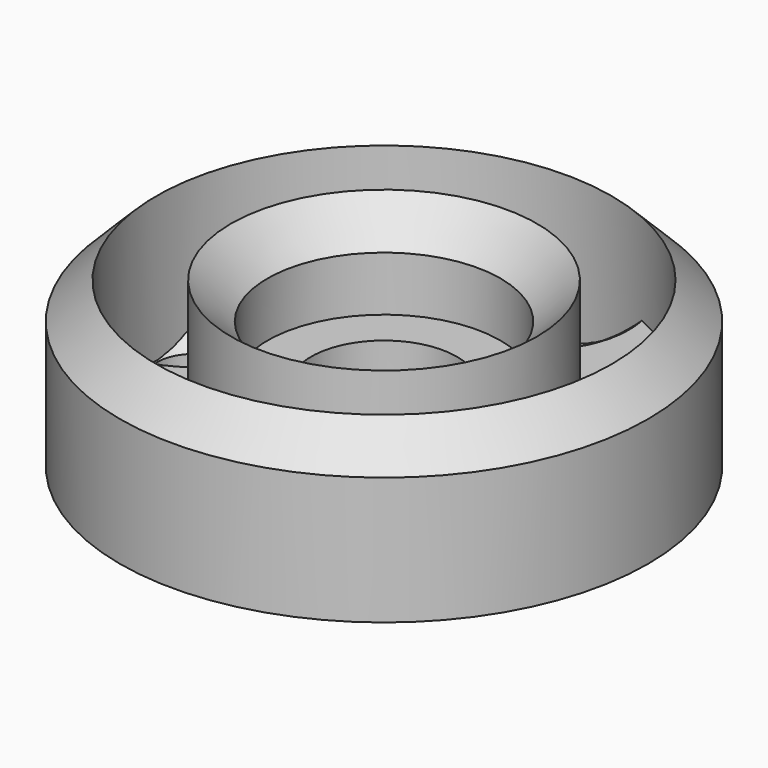
from build123d import *

# Parameters (mm, degrees)
F0_R     = 7.25
F0_R_2   = 6.25
F1_DEPTH = 5
F0_R_3   = 4.2
F0_R_4   = 3.2
F0_R_5   = 2
F2_DEPTH = 2
F0_R_6   = 1


# Not quite as in the source:
# - a fillet or chamfer that OpenCascade refuses, or shapes differently, is made with other operations: its cross-section is extruded or revolved along the edge and cut away or added


with BuildPart() as f1:
    # F0 (on Top) → F1 (new body)
    with BuildSketch(Plane.XY):
        Circle(F0_R)
        Circle(F0_R_2, mode=Mode.SUBTRACT)
    extrude(amount=F1_DEPTH)

    # F3#3: chamfer of 1.5 on 1 edges, made by hand

    # F3_3_s1 → F3_3_t2 (revolve, cut)
    with BuildSketch(Plane.XZ):
        Polygon((7.25, 3.5), (5.75, 5), (7.25, 5), align=None)
    revolve(axis=Axis((0, 0, 5), (0, 0, 1)), mode=Mode.SUBTRACT)


with BuildPart() as f1b:
    # F0 (on Top) → F1, piece 2 (new body)
    with BuildSketch(Plane.XY):
        Circle(F0_R_3)
        Circle(F0_R_4, mode=Mode.SUBTRACT)
    extrude(amount=F1_DEPTH)

    # F3#2: chamfer of 1.5 on 1 edges, made by hand

    # F3_2_s1 → F3_2_t2 (revolve, cut)
    with BuildSketch(Plane.XZ):
        Polygon((3.2, 3.5), (4.7, 5), (3.2, 5), align=None)
    revolve(axis=Axis((0, 0, 5), (0, 0, 1)), mode=Mode.SUBTRACT)


with BuildPart() as f2:
    # F0 (on Top) → F2 (new body)
    with BuildSketch(Plane.XY):
        Circle(F0_R_4)
        Circle(F0_R_5, mode=Mode.SUBTRACT)
    extrude(amount=F2_DEPTH)


with BuildPart() as f2b:
    # F0 (on Top) → F2, piece 2 (new body)
    with BuildSketch(Plane.XY):
        Circle(F0_R_2)
        with Locations((0, -5.2184178494)):
            Circle(F0_R_6, mode=Mode.SUBTRACT)
        with Locations((-5.2160057239, 0)):
            Circle(F0_R_6, mode=Mode.SUBTRACT)
        Circle(F0_R_3, mode=Mode.SUBTRACT)
        with Locations((5.2217580378, 0.0416360635)):
            Circle(F0_R_6, mode=Mode.SUBTRACT)
        with Locations((0.0427705018, 5.2258885844)):
            Circle(F0_R_6, mode=Mode.SUBTRACT)
    extrude(amount=F2_DEPTH)

    # F3: chamfer of 1.5 on 4 edges, made by hand

    # F3_s1 → F3_t2 (revolve, cut)
    with BuildSketch(Plane.XZ):
        Polygon((-4.2160057239, 0.5), (-2.7160057239, 2), (-4.2160057239, 2), align=None)
    revolve(axis=Axis((-5.2160057239, 0, 2), (0, 0, 1)), mode=Mode.SUBTRACT)

    # F3_s3 → F3_t4 (revolve, cut)
    with BuildSketch(Plane.XZ.offset(5.2184178494)):
        Polygon((1, 0.5), (2.5, 2), (1, 2), align=None)
    revolve(axis=Axis((0, -5.2184178494, 2), (0, 0, 1)), mode=Mode.SUBTRACT)

    # F3_s5 → F3_t6 (revolve, cut)
    with BuildSketch(Plane.XZ.offset(-5.2258885844)):
        Polygon((1.0427705018, 0.5), (2.5427705018, 2), (1.0427705018, 2), align=None)
    revolve(axis=Axis((0.0427705018, 5.2258885844, 2), (0, 0, 1)), mode=Mode.SUBTRACT)

    # F3_s7 → F3_t8 (revolve, cut)
    with BuildSketch(Plane.XZ.offset(-0.0416360635)):
        Polygon((6.2217580378, 0.5), (7.7217580378, 2), (6.2217580378, 2), align=None)
    revolve(axis=Axis((5.2217580378, 0.0416360635, 2), (0, 0, 1)), mode=Mode.SUBTRACT)


solid = Compound([f1.part, f1b.part, f2.part, f2b.part])
